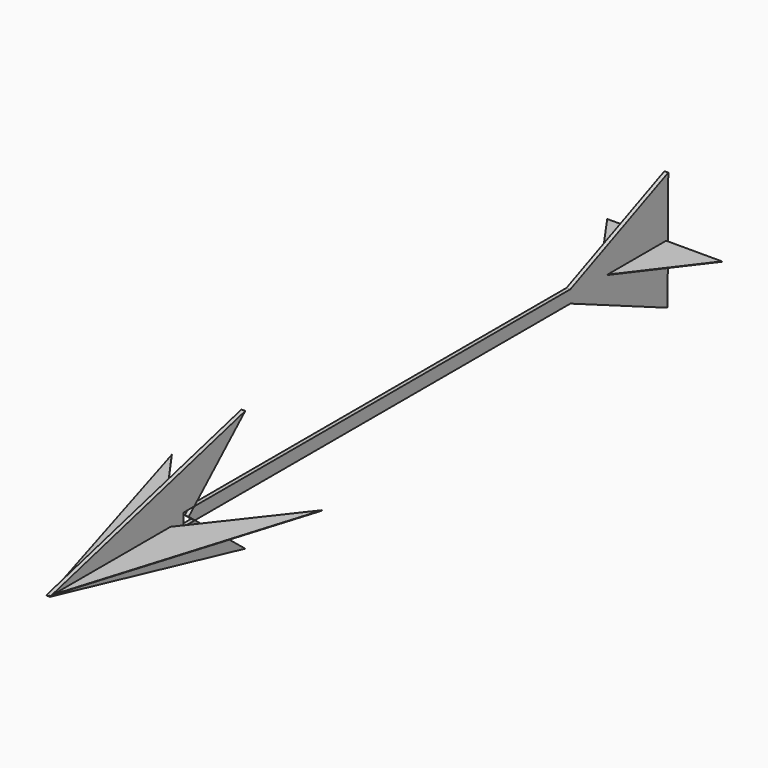
from build123d import *

# Parameters (mm, degrees)
F1_DEPTH = 1
F3_DEPTH = 0.1


# Not quite as in the source:
# - a feature names something its author has since deleted; it is built from what else it names


with BuildPart() as f1:
    # F0 (on Right) → F1 (new body)
    with BuildSketch(Plane.YZ):
        Polygon((62.826286089, -1.6406250652), (62.826286089, 1.6406250652), (-59.3336690074, 1.6406250652), (-61.1351393163, 0), (-59.0934728905, -1.6406250652), align=None)
        Polygon((94.6203459122, 15.4029149351), (62.826286089, 1.6406250652), (62.826286089, -1.6406250652), (94.3906232715, -15.4218757525), align=None)
    extrude(amount=F1_DEPTH)


with BuildPart() as f1b:
    # F0 (on Right) → F1, piece 2 (new body)
    with BuildSketch(Plane.YZ):
        Polygon((-62.826286089, 1.6406250652), (-59.3336690074, 1.6406250652), (-42.7601411939, 16.7343765497), (-106.1958223581, 0), (-62.826286089, 0), align=None)
        Polygon((-42.7601411939, -14.7656258196), (-59.0934728905, -1.6406250652), (-62.826286089, -1.6406250652), (-62.826286089, 0), (-106.1958223581, 0), align=None)
    extrude(amount=F1_DEPTH)


with BuildPart() as f3:
    # F2 (on Top) → F3 (new body)
    with BuildSketch(Plane.XY):
        Polygon((20.4486493021, -42.1203821898), (0, -68.3291633233), (-18.5940028665, -42.1203821898), (0.6650799187, -106.2591299415), align=None)
    extrude(amount=F3_DEPTH)


with BuildPart() as f3b:
    # F2 (on Top) → F3, piece 2 (new body)
    with BuildSketch(Plane.XY):
        Polygon((-14.3123809248, 93.9247533679), (0, 73.5628083348), (15.492782928, 93.9247533679), align=None)
    extrude(amount=F3_DEPTH)


solid = Compound([f1.part, f1b.part, f3.part, f3b.part])
